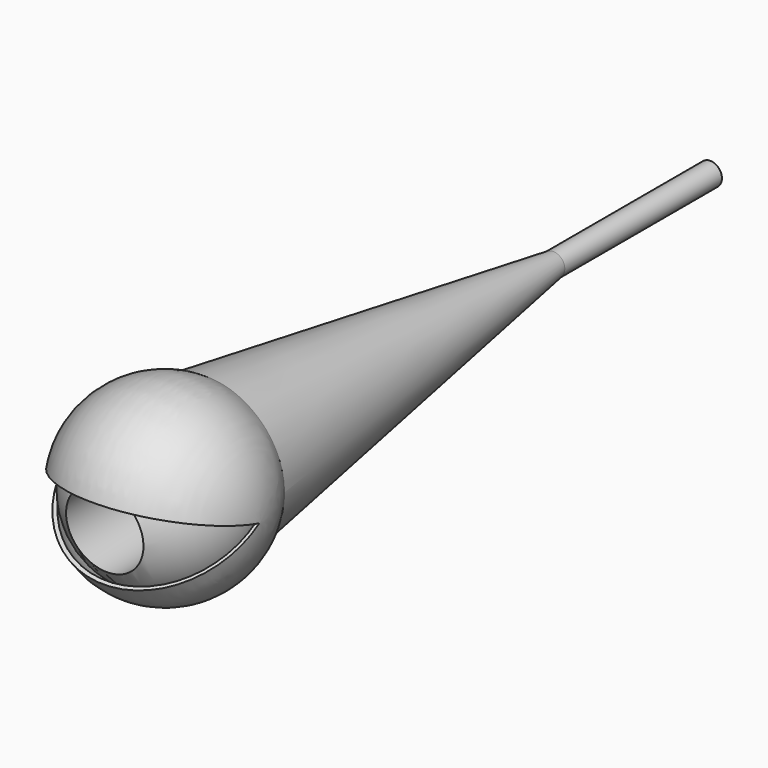
from build123d import *

# Parameters (mm, degrees)
F2_R          = 5
F3_DEPTH      = 11.43
F4_ANGLE_BACK = 75
F4_ANGLE      = 310
F6_R          = 10.5
F8_R          = 1.5
F10_DEPTH     = 25.4
F11_R         = 0.9413311722
F12_DEPTH     = 25.4


with BuildPart() as f1:
    # F0 (on Front) → F1 (revolve)
    with BuildSketch(Plane.XZ):
        with BuildLine():
            Line((0, 0), (11, 0))
            ThreePointArc((11, 0), (0, 11), (-11, 0))
            Line((-11, 0), (0, 0))
        make_face()
    revolve(axis=Axis((0, 0, 0), (1, 0, 0)))

    # F2 (on Front) → F3 (cut)
    with BuildSketch(Plane.XZ):
        with Locations((0, -0.6990660331)):
            Circle(F2_R)
    extrude(amount=F3_DEPTH, mode=Mode.SUBTRACT)


with BuildPart() as f4:
    # F0 (on Front) → F4 (revolve)
    with BuildSketch(Plane.XZ, mode=Mode.PRIVATE) as f4_sk:
        with BuildLine():
            ThreePointArc((-11.7385368794, 0), (0.0044796616, 11.5883666334), (11.7474962026, 0))
            Line((11.7474962026, 0), (12.1738109738, 0))
            ThreePointArc((12.1738109738, 0), (-0.0730315223, 12.0663427521), (-12.3198740184, 0))
            Line((-12.3198740184, 0), (-11.7385368794, 0))
        make_face()
    revolve(f4_sk.sketch.rotate(Axis((0, 0, 0), (-1, 0, 0)), -F4_ANGLE_BACK), axis=Axis((0, 0, 0), (-1, 0, 0)), revolution_arc=F4_ANGLE)

    # F6 (on offset) → F9 section 0
    with BuildSketch(Plane.XZ.offset(-3.1242)):
        Circle(F6_R)
    # F8 (on offset) → F9 section 1
    with BuildSketch(Plane.XZ.offset(-62.738)):
        Circle(F8_R)
    loft()

    # F10 (add): a face of the model
    f10_faces = [f4.faces().sort_by_distance(p)[0] for p in [
        (0, 62.738, 0),
    ]]
    extrude(f10_faces, amount=F10_DEPTH)

    # F11 (on face) → F12 (cut)
    with BuildSketch(Plane(origin=(0, 88.138, 0), x_dir=(-1, 0, 0), z_dir=(0, 1, 0))):
        Circle(F11_R)
    extrude(amount=-F12_DEPTH, mode=Mode.SUBTRACT)


solid = Compound([f1.part, f4.part])
